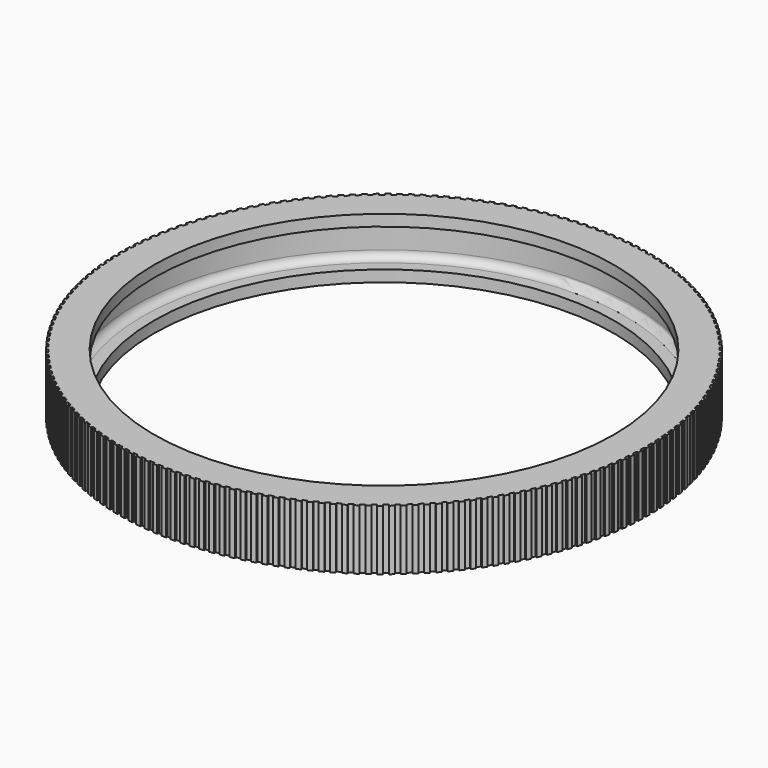
from build123d import *

# Parameters (mm, degrees)
F2_R     = 1
F4_DEPTH = 8


with BuildPart() as f1:
    # F0 (on Front) → F1 (revolve)
    with BuildSketch(Plane.XZ):
        Polygon((35, 8), (30.5, 8), (30.5, 6.5), (33, 6.5), (33, 1.5), (30.5, 1.5), (30.5, 0), (35, 0), align=None)
    revolve(axis=Axis((0, 0, 5), (0, 0, 1)))

    # F2
    f2_edges = [f1.edges().sort_by_distance(p)[0] for p in [
        (-33, 0, 6.5),
        (-33, 0, 1.5),
    ]]
    fillet(f2_edges, radius=F2_R)

    # F3 (on face) → F4 (cut, through all)
    with BuildSketch(Plane.XY.offset(8)):
        with BuildLine():
            Line((0.9096489537, 34.7380920429), (0.9161931908, 34.9880063741))
            ThreePointArc((0.9161931908, 34.9880063741), (0.6108342253, 34.9946693305), (0.3054287424, 34.9986673072))
            Line((0.3054287424, 34.9986673072), (0.3032471086, 34.7486768265))
            ThreePointArc((0.3032471086, 34.7486768265), (0.6064711237, 34.7447074067), (0.9096489537, 34.7380920429))
        make_face()
        with BuildLine():
            Line((2.1214367488, 34.6851842452), (2.1366988837, 34.9347179448))
            ThreePointArc((2.1366988837, 34.9347179448), (1.8317584685, 34.9520337164), (1.5266785578, 34.9666877554))
            Line((1.5266785578, 34.9666877554), (1.5157737109, 34.7169257))
            ThreePointArc((1.5157737109, 34.7169257), (1.8186744794, 34.7023763327), (2.1214367488, 34.6851842452))
        make_face()
        with BuildLine():
            Line((3.3306399001, 34.5900178933), (3.3546013382, 34.8388669429))
            ThreePointArc((3.3546013382, 34.8388669429), (3.0504509962, 34.8668144332), (2.7460683505, 34.8921066807))
            Line((2.7460683505, 34.8921066807), (2.7264535765, 34.6428773472))
            ThreePointArc((2.7264535765, 34.6428773472), (3.0286620605, 34.6177657587), (3.3306399001, 34.5900178933))
        make_face()
        with BuildLine():
            Line((4.5357851796, 34.4527089327), (4.5684167277, 34.7005701481))
            ThreePointArc((4.5684167277, 34.7005701481), (4.2654270192, 34.7391153074), (3.9621124819, 34.7750149487))
            Line((3.9621124819, 34.7750149487), (3.9338116784, 34.5266219848))
            ThreePointArc((3.9338116784, 34.5266219848), (4.2349596833, 34.4909787695), (4.5357851796, 34.4527089327))
        make_face()
        with BuildLine():
            Line((5.7354043037, 34.2734246534), (5.7766662051, 34.5199960538))
            ThreePointArc((5.7766662051, 34.5199960538), (5.4752062764, 34.5690919208), (5.1733293895, 34.6155552177))
            Line((5.1733293895, 34.6155552177), (5.1363770368, 34.3683012518))
            ThreePointArc((5.1363770368, 34.3683012518), (5.4360976601, 34.3221698357), (5.7354043037, 34.2734246534))
        make_face()
        with BuildLine():
            Line((6.928035721, 34.0523834856), (6.9778777046, 34.2973646617))
            ThreePointArc((6.9778777046, 34.2973646617), (6.6783148382, 34.3569514207), (6.3782433922, 34.4139217647))
            Line((6.3782433922, 34.4139217647), (6.3326845109, 34.1681080378))
            ThreePointArc((6.3326845109, 34.1681080378), (6.6306125893, 34.1115446248), (6.928035721, 34.0523834856))
        make_face()
        with BuildLine():
            Line((8.112226394, 33.7898547338), (8.170587735, 34.0329472139))
            ThreePointArc((8.170587735, 34.0329472139), (7.873286902, 34.1029522675), (7.5753864878, 34.1703602492))
            Line((7.5753864878, 34.1703602492), (7.5212765843, 33.9262862474))
            ThreePointArc((7.5212765843, 33.9262862474), (7.8170491384, 33.8593597513), (8.112226394, 33.7898547338))
        make_face()
        with BuildLine():
            Line((9.2865335687, 33.486158249), (9.3533431627, 33.7270658623))
            ThreePointArc((9.3533431627, 33.7270658623), (9.0586665786, 33.8074039201), (8.7633001419, 33.8851674132))
            Line((8.7633001419, 33.8851674132), (8.7007051409, 33.6431305031))
            ThreePointArc((8.7007051409, 33.6431305031), (8.9939618173, 33.5659224635), (9.2865335687, 33.486158249))
        make_face()
        with BuildLine():
            Line((10.4495265328, 33.1416640385), (10.5247029826, 33.3800932762))
            ThreePointArc((10.5247029826, 33.3800932762), (10.2330096653, 33.4706664587), (9.9405370646, 33.5586907204))
            Line((9.9405370646, 33.5586907204), (9.8695332285, 33.3189857867))
            ThreePointArc((9.8695332285, 33.3189857867), (10.1599167391, 33.2315902697), (10.4495265328, 33.1416640385))
        make_face()
        with BuildLine():
            Line((11.5997883584, 32.7567918155), (11.6832400732, 32.9924521882))
            ThreePointArc((11.6832400732, 32.9924521882), (11.394885406, 33.093150146), (11.1056629742, 33.1913279322))
            Line((11.1056629742, 33.1913279322), (11.0263368101, 32.9542470184))
            ThreePointArc((11.0263368101, 32.9542470184), (11.3134933674, 32.8567705021), (11.5997883584, 32.7567918155))
        make_face()
        with BuildLine():
            Line((12.7359176287, 32.3320104874), (12.8275429354, 32.5646148794))
            ThreePointArc((12.8275429354, 32.5646148794), (12.5428782341, 32.6753149274), (12.2572583441, 32.7835266237))
            Line((12.2572583441, 32.7835266237), (12.1697064988, 32.5493585764))
            ThreePointArc((12.1697064988, 32.5493585764), (12.4532862467, 32.4419198208), (12.7359176287, 32.3320104874))
        make_face()
        with BuildLine():
            Line((13.8565301452, 31.8678375849), (13.9562174124, 32.0971026035))
            ThreePointArc((13.9562174124, 32.0971026035), (13.6755894971, 32.2176698708), (13.3939201328, 32.3357836379))
            Line((13.3939201328, 32.3357836379), (13.2982492747, 32.1048137548))
            ThreePointArc((13.2982492747, 32.1048137548), (13.577906715, 31.9875436575), (13.8565301452, 31.8678375849))
        make_face()
        with BuildLine():
            Line((14.9602606141, 31.3648386312), (15.0678883883, 31.5904849522))
            ThreePointArc((15.0678883883, 31.5904849522), (14.7916391609, 31.7207725463), (14.514263493, 31.8486444807))
            Line((14.514263493, 31.8486444807), (14.4105901823, 31.621154163))
            ThreePointArc((14.4105901823, 31.621154163), (14.6859845955, 31.4941955995), (14.9602606141, 31.3648386312))
        make_face()
        with BuildLine():
            Line((16.0457643099, 30.8236264529), (16.1612014632, 31.0453791612))
            ThreePointArc((16.1612014632, 31.0453791612), (15.8896674909, 31.1852283466), (15.6169234588, 31.3227026561))
            Line((15.6169234588, 31.3227026561), (15.5053740056, 31.0989690657))
            ThreePointArc((15.5053740056, 31.0989690657), (15.7761698659, 30.9624767155), (16.0457643099, 30.8236264529))
        make_face()
        with BuildLine():
            Line((17.1117187136, 30.2448604339), (17.2348246036, 30.4624493579))
            ThreePointArc((17.2348246036, 30.4624493579), (16.9683367086, 30.6116897499), (16.7005566091, 30.7585989432))
            Line((16.7005566091, 30.7585989432), (16.581266919, 30.538894665))
            ThreePointArc((16.581266919, 30.538894665), (16.8471343036, 30.3930348231), (17.1117187136, 30.2448604339))
        make_face()
        with BuildLine():
            Line((18.1568251239, 29.6292457113), (18.2874497651, 29.8424057524))
            ThreePointArc((18.2874497651, 29.8424057524), (18.0263326219, 30.0008555246), (17.7638427036, 30.1570206155))
            Line((17.7638427036, 30.1570206155), (17.6369581129, 29.9416133253))
            ThreePointArc((17.6369581129, 29.9416133253), (17.8975731031, 29.7865636994), (18.1568251239, 29.6292457113))
        make_face()
        with BuildLine():
            Line((19.1798102396, 28.9775323168), (19.3177944859, 29.1860037723))
            ThreePointArc((19.3177944859, 29.1860037723), (19.0623662255, 29.3534698781), (18.8054862921, 29.5187006034))
            Line((18.8054862921, 29.5187006034), (18.6711613901, 29.307852742))
            ThreePointArc((18.6711613901, 29.307852742), (18.9262064668, 29.1438022361), (19.1798102396, 28.9775323168))
        make_face()
        with BuildLine():
            Line((20.179427711, 28.2905142629), (20.3246034499, 28.4940431425))
            ThreePointArc((20.3246034499, 28.4940431425), (20.0751752723, 28.6703215501), (19.8242182924, 28.8444166018))
            Line((19.8242182924, 28.8444166018), (19.6826167331, 28.6383850546))
            ThreePointArc((19.6826167331, 28.6383850546), (19.9317811632, 28.465533539), (20.179427711, 28.2905142629))
        make_face()
        with BuildLine():
            Line((21.1544596581, 27.5690285751), (21.3066500153, 27.7673669102))
            ThreePointArc((21.3066500153, 27.7673669102), (21.0635258103, 27.9522428517), (20.8187975363, 28.1349901216))
            Line((20.8187975363, 28.1349901216), (20.6700918396, 27.9340259064))
            ThreePointArc((20.6700918396, 27.9340259064), (20.9130720545, 27.7525839741), (21.1544596581, 27.5690285751))
        make_face()
        with BuildLine():
            Line((22.1037181547, 26.8139542727), (22.2627377097, 27.0068604186))
            ThreePointArc((22.2627377097, 27.0068604186), (22.0262136867, 27.200108651), (21.7880122823, 27.3912854898))
            Line((21.7880122823, 27.3912854898), (21.6323836232, 27.1956334506))
            ThreePointArc((21.6323836232, 27.1956334506), (21.868883589, 27.0058221606), (22.1037181547, 26.8139542727))
        make_face()
        with BuildLine():
            Line((23.0260466755, 26.0262112974), (23.1917016875, 26.2134502276))
            ThreePointArc((23.1917016875, 26.2134502276), (22.9620660147, 26.4148353078), (22.7306816916, 26.614208796))
            Line((22.7306816916, 26.614208796), (22.5683196795, 26.4241073046))
            ThreePointArc((22.5683196795, 26.4241073046), (22.7980512574, 26.2261579127), (23.0260466755, 26.0262112974))
        make_face()
        with BuildLine():
            Line((23.9203215054, 25.2067593927), (24.0924101493, 25.3881029854))
            ThreePointArc((24.0924101493, 25.3881029854), (23.8699426022, 25.5973795567), (23.6456572665, 25.8047067884))
            Line((23.6456572665, 25.8047067884), (23.4767597146, 25.6203874541))
            ThreePointArc((23.4767597146, 25.6203874541), (23.6994430122, 25.4145411313), (23.9203215054, 25.2067593927))
        make_face()
        with BuildLine():
            Line((24.7854531081, 24.3565969344), (24.9637657204, 24.5318242505))
            ThreePointArc((24.9637657204, 24.5318242505), (24.7487373415, 24.7487373415), (24.5318242505, 24.9637657204))
            Line((24.5318242505, 24.9637657204), (24.3565969344, 24.7854531081))
            ThreePointArc((24.3565969344, 24.7854531081), (24.5719606462, 24.5719606462), (24.7854531081, 24.3565969344))
        make_face()
        with BuildLine():
            Line((25.6203874542, 23.4767597146), (25.8047067884, 23.6456572665))
            ThreePointArc((25.8047067884, 23.6456572665), (25.5973795567, 23.8699426022), (25.3881029854, 24.0924101493))
            Line((25.3881029854, 24.0924101493), (25.2067593927, 23.9203215054))
            ThreePointArc((25.2067593927, 23.9203215054), (25.4145411313, 23.6994430122), (25.6203874542, 23.4767597146))
        make_face()
        with BuildLine():
            Line((26.4241073046, 22.5683196795), (26.614208796, 22.7306816916))
            ThreePointArc((26.614208796, 22.7306816916), (26.4148353078, 22.9620660147), (26.2134502276, 23.1917016875))
            Line((26.2134502276, 23.1917016875), (26.0262112974, 23.0260466755))
            ThreePointArc((26.0262112974, 23.0260466755), (26.2261579127, 22.7980512574), (26.4241073046, 22.5683196795))
        make_face()
        with BuildLine():
            Line((27.1956334506, 21.6323836232), (27.3912854898, 21.7880122823))
            ThreePointArc((27.3912854898, 21.7880122823), (27.200108651, 22.0262136867), (27.0068604186, 22.2627377097))
            Line((27.0068604186, 22.2627377097), (26.8139542727, 22.1037181546))
            ThreePointArc((26.8139542727, 22.1037181546), (27.0058221606, 21.868883589), (27.1956334506, 21.6323836232))
        make_face()
        with BuildLine():
            Line((27.9340259064, 20.6700918396), (28.1349901216, 20.8187975363))
            ThreePointArc((28.1349901216, 20.8187975363), (27.9522428517, 21.0635258103), (27.7673669102, 21.3066500153))
            Line((27.7673669102, 21.3066500153), (27.5690285751, 21.154459658))
            ThreePointArc((27.5690285751, 21.154459658), (27.7525839741, 20.9130720545), (27.9340259064, 20.6700918396))
        make_face()
        with BuildLine():
            Line((28.6383850546, 19.6826167331), (28.8444166018, 19.8242182924))
            ThreePointArc((28.8444166018, 19.8242182924), (28.6703215501, 20.0751752723), (28.4940431425, 20.3246034499))
            Line((28.4940431425, 20.3246034499), (28.2905142629, 20.179427711))
            ThreePointArc((28.2905142629, 20.179427711), (28.465533539, 19.9317811632), (28.6383850546, 19.6826167331))
        make_face()
        with BuildLine():
            Line((29.307852742, 18.67116139), (29.5187006034, 18.8054862921))
            ThreePointArc((29.5187006034, 18.8054862921), (29.3534698781, 19.0623662255), (29.1860037723, 19.3177944859))
            Line((29.1860037723, 19.3177944859), (28.9775323168, 19.1798102396))
            ThreePointArc((28.9775323168, 19.1798102396), (29.1438022361, 18.9262064668), (29.307852742, 18.67116139))
        make_face()
        with BuildLine():
            Line((29.9416133253, 17.6369581129), (30.1570206155, 17.7638427036))
            ThreePointArc((30.1570206155, 17.7638427036), (30.0008555246, 18.0263326218), (29.8424057524, 18.2874497651))
            Line((29.8424057524, 18.2874497651), (29.6292457113, 18.1568251239))
            ThreePointArc((29.6292457113, 18.1568251239), (29.7865636994, 17.8975731031), (29.9416133253, 17.6369581129))
        make_face()
        with BuildLine():
            Line((30.538894665, 16.581266919), (30.7585989432, 16.7005566091))
            ThreePointArc((30.7585989432, 16.7005566091), (30.6116897499, 16.9683367086), (30.4624493579, 17.2348246036))
            Line((30.4624493579, 17.2348246036), (30.2448604339, 17.1117187136))
            ThreePointArc((30.2448604339, 17.1117187136), (30.3930348231, 16.8471343036), (30.538894665, 16.581266919))
        make_face()
        with BuildLine():
            Line((31.0989690657, 15.5053740056), (31.3227026561, 15.6169234588))
            ThreePointArc((31.3227026561, 15.6169234588), (31.1852283466, 15.8896674909), (31.0453791612, 16.1612014632))
            Line((31.0453791612, 16.1612014632), (30.8236264529, 16.0457643099))
            ThreePointArc((30.8236264529, 16.0457643099), (30.9624767155, 15.7761698659), (31.0989690657, 15.5053740056))
        make_face()
        with BuildLine():
            Line((31.621154163, 14.4105901823), (31.8486444807, 14.514263493))
            ThreePointArc((31.8486444807, 14.514263493), (31.7207725463, 14.7916391609), (31.5904849522, 15.0678883883))
            Line((31.5904849522, 15.0678883883), (31.3648386312, 14.9602606141))
            ThreePointArc((31.3648386312, 14.9602606141), (31.4941955995, 14.6859845955), (31.621154163, 14.4105901823))
        make_face()
        with BuildLine():
            Line((32.1048137548, 13.2982492747), (32.3357836379, 13.3939201328))
            ThreePointArc((32.3357836379, 13.3939201328), (32.2176698708, 13.6755894971), (32.0971026035, 13.9562174124))
            Line((32.0971026035, 13.9562174124), (31.8678375849, 13.8565301451))
            ThreePointArc((31.8678375849, 13.8565301451), (31.9875436575, 13.577906715), (32.1048137548, 13.2982492747))
        make_face()
        with BuildLine():
            Line((32.5493585764, 12.1697064988), (32.7835266237, 12.2572583441))
            ThreePointArc((32.7835266237, 12.2572583441), (32.6753149274, 12.5428782341), (32.5646148794, 12.8275429353))
            Line((32.5646148794, 12.8275429353), (32.3320104874, 12.7359176287))
            ThreePointArc((32.3320104874, 12.7359176287), (32.4419198208, 12.4532862467), (32.5493585764, 12.1697064988))
        make_face()
        with BuildLine():
            Line((32.9542470184, 11.0263368101), (33.1913279322, 11.1056629742))
            ThreePointArc((33.1913279322, 11.1056629742), (33.093150146, 11.394885406), (32.9924521882, 11.6832400732))
            Line((32.9924521882, 11.6832400732), (32.7567918155, 11.5997883584))
            ThreePointArc((32.7567918155, 11.5997883584), (32.8567705021, 11.3134933674), (32.9542470184, 11.0263368101))
        make_face()
        with BuildLine():
            Line((33.3189857867, 9.8695332285), (33.5586907204, 9.9405370646))
            ThreePointArc((33.5586907204, 9.9405370646), (33.4706664587, 10.2330096653), (33.3800932762, 10.5247029826))
            Line((33.3800932762, 10.5247029826), (33.1416640385, 10.4495265328))
            ThreePointArc((33.1416640385, 10.4495265328), (33.2315902697, 10.1599167391), (33.3189857867, 9.8695332285))
        make_face()
        with BuildLine():
            Line((33.6431305031, 8.7007051409), (33.8851674132, 8.7633001419))
            ThreePointArc((33.8851674132, 8.7633001419), (33.8074039201, 9.0586665786), (33.7270658623, 9.3533431627))
            Line((33.7270658623, 9.3533431627), (33.486158249, 9.2865335687))
            ThreePointArc((33.486158249, 9.2865335687), (33.5659224635, 8.9939618173), (33.6431305031, 8.7007051409))
        make_face()
        with BuildLine():
            Line((33.9262862474, 7.5212765843), (34.1703602492, 7.5753864878))
            ThreePointArc((34.1703602492, 7.5753864878), (34.1029522675, 7.873286902), (34.0329472139, 8.170587735))
            Line((34.0329472139, 8.170587735), (33.7898547338, 8.112226394))
            ThreePointArc((33.7898547338, 8.112226394), (33.8593597513, 7.8170491384), (33.9262862474, 7.5212765843))
        make_face()
        with BuildLine():
            Line((34.1681080378, 6.3326845108), (34.4139217647, 6.3782433922))
            ThreePointArc((34.4139217647, 6.3782433922), (34.3569514207, 6.6783148382), (34.2973646617, 6.9778777046))
            Line((34.2973646617, 6.9778777046), (34.0523834856, 6.928035721))
            ThreePointArc((34.0523834856, 6.928035721), (34.1115446248, 6.6306125893), (34.1681080378, 6.3326845108))
        make_face()
        with BuildLine():
            Line((34.3683012518, 5.1363770367), (34.6155552177, 5.1733293895))
            ThreePointArc((34.6155552177, 5.1733293895), (34.5690919208, 5.4752062764), (34.5199960538, 5.7766662051))
            Line((34.5199960538, 5.7766662051), (34.2734246534, 5.7354043037))
            ThreePointArc((34.2734246534, 5.7354043037), (34.3221698357, 5.4360976601), (34.3683012518, 5.1363770367))
        make_face()
        with BuildLine():
            Line((34.5266219848, 3.9338116784), (34.7750149487, 3.9621124819))
            ThreePointArc((34.7750149487, 3.9621124819), (34.7391153074, 4.2654270192), (34.7005701481, 4.5684167277))
            Line((34.7005701481, 4.5684167277), (34.4527089327, 4.5357851796))
            ThreePointArc((34.4527089327, 4.5357851796), (34.4909787695, 4.2349596833), (34.5266219848, 3.9338116784))
        make_face()
        with BuildLine():
            Line((34.6428773472, 2.7264535765), (34.8921066807, 2.7460683505))
            ThreePointArc((34.8921066807, 2.7460683505), (34.8668144332, 3.0504509962), (34.8388669428, 3.3546013382))
            Line((34.8388669428, 3.3546013382), (34.5900178933, 3.3306399001))
            ThreePointArc((34.5900178933, 3.3306399001), (34.6177657587, 3.0286620605), (34.6428773472, 2.7264535765))
        make_face()
        with BuildLine():
            Line((34.7169257, 1.5157737109), (34.9666877554, 1.5266785578))
            ThreePointArc((34.9666877554, 1.5266785578), (34.9520337164, 1.8317584685), (34.9347179448, 2.1366988837))
            Line((34.9347179448, 2.1366988837), (34.6851842452, 2.1214367488))
            ThreePointArc((34.6851842452, 2.1214367488), (34.7023763327, 1.8186744794), (34.7169257, 1.5157737109))
        make_face()
        with BuildLine():
            Line((34.7486768265, 0.3032471086), (34.9986673072, 0.3054287424))
            ThreePointArc((34.9986673072, 0.3054287424), (34.9946693305, 0.6108342253), (34.9880063741, 0.9161931908))
            Line((34.9880063741, 0.9161931908), (34.7380920429, 0.9096489537))
            ThreePointArc((34.7380920429, 0.9096489537), (34.7447074067, 0.6064711237), (34.7486768265, 0.3032471086))
        make_face()
        with BuildLine():
            Line((34.7380920429, -0.9096489537), (34.9880063741, -0.9161931908))
            ThreePointArc((34.9880063741, -0.9161931908), (34.9946693305, -0.6108342253), (34.9986673072, -0.3054287424))
            Line((34.9986673072, -0.3054287424), (34.7486768265, -0.3032471086))
            ThreePointArc((34.7486768265, -0.3032471086), (34.7447074067, -0.6064711237), (34.7380920429, -0.9096489537))
        make_face()
        with BuildLine():
            Line((34.6851842452, -2.1214367488), (34.9347179448, -2.1366988837))
            ThreePointArc((34.9347179448, -2.1366988837), (34.9520337164, -1.8317584685), (34.9666877554, -1.5266785578))
            Line((34.9666877554, -1.5266785578), (34.7169257, -1.515773711))
            ThreePointArc((34.7169257, -1.5157737109), (34.7023763327, -1.8186744794), (34.6851842452, -2.1214367488))
        make_face()
        with BuildLine():
            Line((34.5900178933, -3.3306399001), (34.8388669428, -3.3546013382))
            ThreePointArc((34.8388669428, -3.3546013382), (34.8668144332, -3.0504509962), (34.8921066807, -2.7460683505))
            Line((34.8921066807, -2.7460683505), (34.6428773472, -2.7264535765))
            ThreePointArc((34.6428773472, -2.7264535765), (34.6177657587, -3.0286620605), (34.5900178933, -3.3306399001))
        make_face()
        with BuildLine():
            Line((34.4527089327, -4.5357851797), (34.7005701481, -4.5684167277))
            ThreePointArc((34.7005701481, -4.5684167277), (34.7391153074, -4.2654270192), (34.7750149487, -3.9621124819))
            Line((34.7750149487, -3.9621124819), (34.5266219848, -3.9338116784))
            ThreePointArc((34.5266219848, -3.9338116784), (34.4909787695, -4.2349596833), (34.4527089327, -4.5357851797))
        make_face()
        with BuildLine():
            Line((34.2734246534, -5.7354043037), (34.5199960538, -5.7766662051))
            ThreePointArc((34.5199960538, -5.7766662051), (34.5690919208, -5.4752062764), (34.6155552177, -5.1733293895))
            Line((34.6155552177, -5.1733293895), (34.3683012518, -5.1363770368))
            ThreePointArc((34.3683012518, -5.1363770368), (34.3221698357, -5.4360976602), (34.2734246534, -5.7354043037))
        make_face()
        with BuildLine():
            Line((34.0523834856, -6.928035721), (34.2973646617, -6.9778777046))
            ThreePointArc((34.2973646617, -6.9778777046), (34.3569514207, -6.6783148382), (34.4139217647, -6.3782433922))
            Line((34.4139217647, -6.3782433922), (34.1681080378, -6.3326845109))
            ThreePointArc((34.1681080378, -6.3326845109), (34.1115446248, -6.6306125893), (34.0523834856, -6.928035721))
        make_face()
        with BuildLine():
            Line((33.7898547338, -8.112226394), (34.0329472139, -8.170587735))
            ThreePointArc((34.0329472139, -8.170587735), (34.1029522675, -7.873286902), (34.1703602492, -7.5753864878))
            Line((34.1703602492, -7.5753864878), (33.9262862474, -7.5212765844))
            ThreePointArc((33.9262862474, -7.5212765844), (33.8593597513, -7.8170491385), (33.7898547338, -8.112226394))
        make_face()
        with BuildLine():
            Line((33.486158249, -9.2865335687), (33.7270658623, -9.3533431627))
            ThreePointArc((33.7270658623, -9.3533431627), (33.8074039201, -9.0586665786), (33.8851674132, -8.7633001419))
            Line((33.8851674132, -8.7633001419), (33.6431305031, -8.7007051409))
            ThreePointArc((33.6431305031, -8.7007051409), (33.5659224635, -8.9939618173), (33.486158249, -9.2865335687))
        make_face()
        with BuildLine():
            Line((33.1416640385, -10.4495265328), (33.3800932762, -10.5247029827))
            ThreePointArc((33.3800932762, -10.5247029827), (33.4706664587, -10.2330096653), (33.5586907204, -9.9405370646))
            Line((33.5586907204, -9.9405370646), (33.3189857867, -9.8695332285))
            ThreePointArc((33.3189857867, -9.8695332285), (33.2315902697, -10.1599167391), (33.1416640385, -10.4495265328))
        make_face()
        with BuildLine():
            Line((32.7567918154, -11.5997883584), (32.9924521882, -11.6832400732))
            ThreePointArc((32.9924521882, -11.6832400732), (33.093150146, -11.394885406), (33.1913279322, -11.1056629742))
            Line((33.1913279322, -11.1056629742), (32.9542470184, -11.0263368101))
            ThreePointArc((32.9542470184, -11.0263368101), (32.8567705021, -11.3134933674), (32.7567918154, -11.5997883584))
        make_face()
        with BuildLine():
            Line((32.3320104874, -12.7359176287), (32.5646148794, -12.8275429354))
            ThreePointArc((32.5646148794, -12.8275429354), (32.6753149274, -12.5428782341), (32.7835266237, -12.2572583441))
            Line((32.7835266237, -12.2572583441), (32.5493585764, -12.1697064988))
            ThreePointArc((32.5493585764, -12.1697064988), (32.4419198208, -12.4532862467), (32.3320104874, -12.7359176287))
        make_face()
        with BuildLine():
            Line((31.8678375849, -13.8565301452), (32.0971026035, -13.9562174124))
            ThreePointArc((32.0971026035, -13.9562174124), (32.2176698708, -13.6755894971), (32.3357836379, -13.3939201328))
            Line((32.3357836379, -13.3939201328), (32.1048137548, -13.2982492747))
            ThreePointArc((32.1048137548, -13.2982492747), (31.9875436575, -13.577906715), (31.8678375849, -13.8565301452))
        make_face()
        with BuildLine():
            Line((31.3648386312, -14.9602606141), (31.5904849522, -15.0678883883))
            ThreePointArc((31.5904849522, -15.0678883883), (31.7207725463, -14.7916391609), (31.8486444807, -14.514263493))
            Line((31.8486444807, -14.514263493), (31.621154163, -14.4105901823))
            ThreePointArc((31.621154163, -14.4105901823), (31.4941955995, -14.6859845955), (31.3648386312, -14.9602606141))
        make_face()
        with BuildLine():
            Line((30.8236264529, -16.0457643099), (31.0453791612, -16.1612014632))
            ThreePointArc((31.0453791612, -16.1612014632), (31.1852283466, -15.8896674909), (31.3227026561, -15.6169234588))
            Line((31.3227026561, -15.6169234588), (31.0989690657, -15.5053740056))
            ThreePointArc((31.0989690657, -15.5053740056), (30.9624767155, -15.776169866), (30.8236264529, -16.0457643099))
        make_face()
        with BuildLine():
            Line((30.2448604339, -17.1117187136), (30.4624493579, -17.2348246036))
            ThreePointArc((30.4624493579, -17.2348246036), (30.6116897499, -16.9683367086), (30.7585989432, -16.7005566091))
            Line((30.7585989432, -16.7005566091), (30.538894665, -16.581266919))
            ThreePointArc((30.538894665, -16.581266919), (30.3930348231, -16.8471343036), (30.2448604339, -17.1117187136))
        make_face()
        with BuildLine():
            Line((29.6292457113, -18.1568251239), (29.8424057524, -18.2874497651))
            ThreePointArc((29.8424057524, -18.2874497651), (30.0008555246, -18.0263326219), (30.1570206154, -17.7638427036))
            Line((30.1570206154, -17.7638427036), (29.9416133253, -17.6369581129))
            ThreePointArc((29.9416133253, -17.6369581129), (29.7865636994, -17.8975731031), (29.6292457113, -18.1568251239))
        make_face()
        with BuildLine():
            Line((28.9775323168, -19.1798102396), (29.1860037723, -19.3177944859))
            ThreePointArc((29.1860037723, -19.3177944859), (29.3534698781, -19.0623662255), (29.5187006034, -18.8054862921))
            Line((29.5187006034, -18.8054862921), (29.307852742, -18.6711613901))
            ThreePointArc((29.307852742, -18.6711613901), (29.1438022361, -18.9262064668), (28.9775323168, -19.1798102396))
        make_face()
        with BuildLine():
            Line((28.2905142629, -20.179427711), (28.4940431425, -20.3246034499))
            ThreePointArc((28.4940431425, -20.3246034499), (28.6703215501, -20.0751752723), (28.8444166018, -19.8242182924))
            Line((28.8444166018, -19.8242182924), (28.6383850546, -19.6826167331))
            ThreePointArc((28.6383850546, -19.6826167331), (28.465533539, -19.9317811632), (28.2905142629, -20.179427711))
        make_face()
        with BuildLine():
            Line((27.5690285751, -21.1544596581), (27.7673669102, -21.3066500153))
            ThreePointArc((27.7673669102, -21.3066500153), (27.9522428516, -21.0635258103), (28.1349901216, -20.8187975363))
            Line((28.1349901216, -20.8187975363), (27.9340259064, -20.6700918396))
            ThreePointArc((27.9340259064, -20.6700918396), (27.7525839741, -20.9130720545), (27.5690285751, -21.1544596581))
        make_face()
        with BuildLine():
            Line((26.8139542727, -22.1037181547), (27.0068604186, -22.2627377097))
            ThreePointArc((27.0068604186, -22.2627377097), (27.200108651, -22.0262136867), (27.3912854898, -21.7880122823))
            Line((27.3912854898, -21.7880122823), (27.1956334506, -21.6323836232))
            ThreePointArc((27.1956334506, -21.6323836232), (27.0058221606, -21.868883589), (26.8139542727, -22.1037181547))
        make_face()
        with BuildLine():
            Line((26.0262112974, -23.0260466755), (26.2134502276, -23.1917016876))
            ThreePointArc((26.2134502276, -23.1917016876), (26.4148353078, -22.9620660147), (26.614208796, -22.7306816916))
            Line((26.614208796, -22.7306816916), (26.4241073046, -22.5683196795))
            ThreePointArc((26.4241073046, -22.5683196795), (26.2261579127, -22.7980512574), (26.0262112974, -23.0260466755))
        make_face()
        with BuildLine():
            Line((25.2067593927, -23.9203215054), (25.3881029854, -24.0924101493))
            ThreePointArc((25.3881029854, -24.0924101493), (25.5973795567, -23.8699426022), (25.8047067883, -23.6456572666))
            Line((25.8047067883, -23.6456572666), (25.6203874541, -23.4767597146))
            ThreePointArc((25.6203874541, -23.4767597146), (25.4145411313, -23.6994430122), (25.2067593927, -23.9203215054))
        make_face()
        with BuildLine():
            Line((24.3565969344, -24.7854531081), (24.5318242505, -24.9637657204))
            ThreePointArc((24.5318242505, -24.9637657204), (24.7487373415, -24.7487373415), (24.9637657204, -24.5318242505))
            Line((24.9637657204, -24.5318242505), (24.7854531081, -24.3565969344))
            ThreePointArc((24.7854531081, -24.3565969344), (24.5719606462, -24.5719606462), (24.3565969344, -24.7854531081))
        make_face()
        with BuildLine():
            Line((23.4767597146, -25.6203874542), (23.6456572665, -25.8047067884))
            ThreePointArc((23.6456572665, -25.8047067884), (23.8699426022, -25.5973795567), (24.0924101493, -25.3881029854))
            Line((24.0924101493, -25.3881029854), (23.9203215053, -25.2067593927))
            ThreePointArc((23.9203215054, -25.2067593927), (23.6994430122, -25.4145411313), (23.4767597146, -25.6203874542))
        make_face()
        with BuildLine():
            Line((22.5683196795, -26.4241073046), (22.7306816915, -26.614208796))
            ThreePointArc((22.7306816915, -26.614208796), (22.9620660147, -26.4148353078), (23.1917016875, -26.2134502276))
            Line((23.1917016875, -26.2134502276), (23.0260466755, -26.0262112974))
            ThreePointArc((23.0260466755, -26.0262112974), (22.7980512574, -26.2261579127), (22.5683196795, -26.4241073046))
        make_face()
        with BuildLine():
            Line((21.6323836231, -27.1956334506), (21.7880122823, -27.3912854898))
            ThreePointArc((21.7880122823, -27.3912854898), (22.0262136867, -27.200108651), (22.2627377097, -27.0068604186))
            Line((22.2627377097, -27.0068604186), (22.1037181546, -26.8139542727))
            ThreePointArc((22.1037181546, -26.8139542727), (21.868883589, -27.0058221606), (21.6323836231, -27.1956334506))
        make_face()
        with BuildLine():
            Line((20.6700918396, -27.9340259065), (20.8187975363, -28.1349901216))
            ThreePointArc((20.8187975363, -28.1349901216), (21.0635258103, -27.9522428517), (21.3066500153, -27.7673669102))
            Line((21.3066500153, -27.7673669102), (21.154459658, -27.5690285751))
            ThreePointArc((21.154459658, -27.5690285751), (20.9130720545, -27.7525839741), (20.6700918396, -27.9340259065))
        make_face()
        with BuildLine():
            Line((19.6826167331, -28.6383850546), (19.8242182924, -28.8444166018))
            ThreePointArc((19.8242182924, -28.8444166018), (20.0751752723, -28.6703215501), (20.3246034499, -28.4940431425))
            Line((20.3246034499, -28.4940431425), (20.1794277109, -28.2905142629))
            ThreePointArc((20.1794277109, -28.2905142629), (19.9317811632, -28.465533539), (19.6826167331, -28.6383850546))
        make_face()
        with BuildLine():
            Line((18.67116139, -29.307852742), (18.8054862921, -29.5187006035))
            ThreePointArc((18.8054862921, -29.5187006035), (19.0623662255, -29.3534698781), (19.3177944859, -29.1860037724))
            Line((19.3177944859, -29.1860037724), (19.1798102396, -28.9775323168))
            ThreePointArc((19.1798102396, -28.9775323168), (18.9262064668, -29.1438022361), (18.67116139, -29.307852742))
        make_face()
        with BuildLine():
            Line((17.6369581129, -29.9416133253), (17.7638427036, -30.1570206155))
            ThreePointArc((17.7638427036, -30.1570206155), (18.0263326218, -30.0008555246), (18.2874497651, -29.8424057524))
            Line((18.287449765, -29.8424057524), (18.1568251239, -29.6292457113))
            ThreePointArc((18.1568251239, -29.6292457113), (17.8975731031, -29.7865636994), (17.6369581129, -29.9416133253))
        make_face()
        with BuildLine():
            Line((16.581266919, -30.538894665), (16.7005566091, -30.7585989432))
            ThreePointArc((16.7005566091, -30.7585989432), (16.9683367086, -30.6116897499), (17.2348246036, -30.4624493579))
            Line((17.2348246036, -30.4624493579), (17.1117187136, -30.2448604339))
            ThreePointArc((17.1117187136, -30.2448604339), (16.8471343036, -30.3930348231), (16.581266919, -30.538894665))
        make_face()
        with BuildLine():
            Line((15.5053740056, -31.0989690657), (15.6169234588, -31.3227026561))
            ThreePointArc((15.6169234588, -31.3227026561), (15.8896674909, -31.1852283466), (16.1612014632, -31.0453791612))
            Line((16.1612014632, -31.0453791612), (16.0457643099, -30.8236264529))
            ThreePointArc((16.0457643099, -30.8236264529), (15.7761698659, -30.9624767155), (15.5053740056, -31.0989690657))
        make_face()
        with BuildLine():
            Line((14.4105901823, -31.621154163), (14.514263493, -31.8486444807))
            ThreePointArc((14.514263493, -31.8486444807), (14.7916391609, -31.7207725463), (15.0678883883, -31.5904849522))
            Line((15.0678883883, -31.5904849522), (14.9602606141, -31.3648386312))
            ThreePointArc((14.9602606141, -31.3648386312), (14.6859845955, -31.4941955995), (14.4105901823, -31.621154163))
        make_face()
        with BuildLine():
            Line((13.2982492747, -32.1048137548), (13.3939201328, -32.3357836379))
            ThreePointArc((13.3939201328, -32.3357836379), (13.6755894971, -32.2176698708), (13.9562174124, -32.0971026035))
            Line((13.9562174124, -32.0971026035), (13.8565301451, -31.8678375849))
            ThreePointArc((13.8565301451, -31.8678375849), (13.577906715, -31.9875436575), (13.2982492747, -32.1048137548))
        make_face()
        with BuildLine():
            Line((12.1697064988, -32.5493585764), (12.2572583441, -32.7835266237))
            ThreePointArc((12.2572583441, -32.7835266237), (12.5428782341, -32.6753149274), (12.8275429353, -32.5646148794))
            Line((12.8275429353, -32.5646148794), (12.7359176287, -32.3320104874))
            ThreePointArc((12.7359176287, -32.3320104874), (12.4532862467, -32.4419198208), (12.1697064988, -32.5493585764))
        make_face()
        with BuildLine():
            Line((11.0263368101, -32.9542470184), (11.1056629742, -33.1913279322))
            ThreePointArc((11.1056629742, -33.1913279322), (11.394885406, -33.093150146), (11.6832400732, -32.9924521882))
            Line((11.6832400732, -32.9924521882), (11.5997883584, -32.7567918155))
            ThreePointArc((11.5997883584, -32.7567918155), (11.3134933674, -32.8567705021), (11.0263368101, -32.9542470184))
        make_face()
        with BuildLine():
            Line((9.8695332285, -33.3189857867), (9.9405370646, -33.5586907204))
            ThreePointArc((9.9405370646, -33.5586907204), (10.2330096653, -33.4706664587), (10.5247029826, -33.3800932762))
            Line((10.5247029826, -33.3800932762), (10.4495265328, -33.1416640385))
            ThreePointArc((10.4495265328, -33.1416640385), (10.1599167391, -33.2315902697), (9.8695332285, -33.3189857867))
        make_face()
        with BuildLine():
            Line((8.7007051409, -33.6431305031), (8.7633001419, -33.8851674132))
            ThreePointArc((8.7633001419, -33.8851674132), (9.0586665786, -33.8074039201), (9.3533431627, -33.7270658623))
            Line((9.3533431627, -33.7270658623), (9.2865335687, -33.486158249))
            ThreePointArc((9.2865335687, -33.486158249), (8.9939618173, -33.5659224635), (8.7007051409, -33.6431305031))
        make_face()
        with BuildLine():
            Line((7.5212765843, -33.9262862474), (7.5753864878, -34.1703602492))
            ThreePointArc((7.5753864878, -34.1703602492), (7.873286902, -34.1029522675), (8.1705877349, -34.0329472139))
            Line((8.1705877349, -34.0329472139), (8.112226394, -33.7898547338))
            ThreePointArc((8.112226394, -33.7898547338), (7.8170491384, -33.8593597513), (7.5212765843, -33.9262862474))
        make_face()
        with BuildLine():
            Line((6.3326845108, -34.1681080378), (6.3782433922, -34.4139217647))
            ThreePointArc((6.3782433922, -34.4139217647), (6.6783148382, -34.3569514207), (6.9778777046, -34.2973646617))
            Line((6.9778777046, -34.2973646617), (6.928035721, -34.0523834856))
            ThreePointArc((6.928035721, -34.0523834856), (6.6306125893, -34.1115446248), (6.3326845108, -34.1681080378))
        make_face()
        with BuildLine():
            Line((5.1363770367, -34.3683012518), (5.1733293895, -34.6155552177))
            ThreePointArc((5.1733293895, -34.6155552177), (5.4752062764, -34.5690919208), (5.7766662051, -34.5199960538))
            Line((5.7766662051, -34.5199960538), (5.7354043036, -34.2734246534))
            ThreePointArc((5.7354043036, -34.2734246534), (5.4360976601, -34.3221698357), (5.1363770367, -34.3683012518))
        make_face()
        with BuildLine():
            Line((3.9338116784, -34.5266219848), (3.9621124819, -34.7750149487))
            ThreePointArc((3.9621124819, -34.7750149487), (4.2654270192, -34.7391153074), (4.5684167277, -34.7005701481))
            Line((4.5684167277, -34.7005701481), (4.5357851796, -34.4527089327))
            ThreePointArc((4.5357851796, -34.4527089327), (4.2349596833, -34.4909787695), (3.9338116784, -34.5266219848))
        make_face()
        with BuildLine():
            Line((2.7264535765, -34.6428773472), (2.7460683505, -34.8921066807))
            ThreePointArc((2.7460683505, -34.8921066807), (3.0504509962, -34.8668144332), (3.3546013382, -34.8388669429))
            Line((3.3546013382, -34.8388669429), (3.3306399001, -34.5900178933))
            ThreePointArc((3.3306399001, -34.5900178933), (3.0286620605, -34.6177657587), (2.7264535765, -34.6428773472))
        make_face()
        with BuildLine():
            Line((1.5157737109, -34.7169257), (1.5266785578, -34.9666877554))
            ThreePointArc((1.5266785578, -34.9666877554), (1.8317584685, -34.9520337164), (2.1366988837, -34.9347179448))
            Line((2.1366988837, -34.9347179448), (2.1214367488, -34.6851842452))
            ThreePointArc((2.1214367488, -34.6851842452), (1.8186744794, -34.7023763327), (1.5157737109, -34.7169257))
        make_face()
        with BuildLine():
            Line((0.3032471086, -34.7486768265), (0.3054287424, -34.9986673072))
            ThreePointArc((0.3054287424, -34.9986673072), (0.6108342253, -34.9946693305), (0.9161931908, -34.9880063741))
            Line((0.9161931908, -34.9880063741), (0.9096489537, -34.7380920429))
            ThreePointArc((0.9096489537, -34.7380920429), (0.6064711237, -34.7447074067), (0.3032471086, -34.7486768265))
        make_face()
        with BuildLine():
            ThreePointArc((-34.9880063741, 0.9161931908), (-34.9946693305, 0.6108342253), (-34.9986673072, 0.3054287424))
            Line((-34.9986673072, 0.3054287424), (-34.7486768265, 0.3032471086))
            ThreePointArc((-34.7486768265, 0.3032471086), (-34.7447074067, 0.6064711237), (-34.7380920429, 0.9096489537))
            Line((-34.7380920429, 0.9096489537), (-34.9880063741, 0.9161931908))
        make_face()
        with BuildLine():
            ThreePointArc((-34.9347179448, 2.1366988837), (-34.9520337164, 1.8317584685), (-34.9666877554, 1.5266785578))
            Line((-34.9666877554, 1.5266785578), (-34.7169257, 1.5157737109))
            ThreePointArc((-34.7169257, 1.5157737109), (-34.7023763327, 1.8186744794), (-34.6851842452, 2.1214367488))
            Line((-34.6851842452, 2.1214367488), (-34.9347179448, 2.1366988837))
        make_face()
        with BuildLine():
            ThreePointArc((-34.8388669428, 3.3546013382), (-34.8668144332, 3.0504509962), (-34.8921066807, 2.7460683505))
            Line((-34.8921066807, 2.7460683505), (-34.6428773472, 2.7264535765))
            ThreePointArc((-34.6428773472, 2.7264535765), (-34.6177657587, 3.0286620605), (-34.5900178933, 3.3306399001))
            Line((-34.5900178933, 3.3306399001), (-34.8388669428, 3.3546013382))
        make_face()
        with BuildLine():
            ThreePointArc((-34.9986673072, -0.3054287424), (-34.9946693305, -0.6108342253), (-34.9880063741, -0.9161931908))
            Line((-34.9880063741, -0.9161931908), (-34.7380920429, -0.9096489537))
            ThreePointArc((-34.7380920429, -0.9096489537), (-34.7447074067, -0.6064711237), (-34.7486768265, -0.3032471086))
            Line((-34.7486768265, -0.3032471086), (-34.9986673072, -0.3054287424))
        make_face()
        with BuildLine():
            Line((-34.7169257, -1.515773711), (-34.9666877554, -1.5266785578))
            ThreePointArc((-34.9666877554, -1.5266785578), (-34.9520337164, -1.8317584685), (-34.9347179448, -2.1366988837))
            Line((-34.9347179448, -2.1366988837), (-34.6851842452, -2.1214367488))
            ThreePointArc((-34.6851842452, -2.1214367488), (-34.7023763327, -1.8186744794), (-34.7169257, -1.5157737109))
        make_face()
        with BuildLine():
            ThreePointArc((-6.3782433922, 34.4139217647), (-6.6783148382, 34.3569514207), (-6.9778777046, 34.2973646617))
            Line((-6.9778777046, 34.2973646617), (-6.928035721, 34.0523834856))
            ThreePointArc((-6.928035721, 34.0523834856), (-6.6306125893, 34.1115446248), (-6.3326845109, 34.1681080378))
            Line((-6.3326845109, 34.1681080378), (-6.3782433922, 34.4139217647))
        make_face()
        with BuildLine():
            ThreePointArc((-5.1733293895, 34.6155552177), (-5.4752062764, 34.5690919208), (-5.7766662051, 34.5199960538))
            Line((-5.7766662051, 34.5199960538), (-5.7354043037, 34.2734246534))
            ThreePointArc((-5.7354043037, 34.2734246534), (-5.4360976601, 34.3221698357), (-5.1363770368, 34.3683012518))
            Line((-5.1363770368, 34.3683012518), (-5.1733293895, 34.6155552177))
        make_face()
        with BuildLine():
            Line((-2.7264535765, 34.6428773472), (-2.7460683505, 34.8921066807))
            ThreePointArc((-2.7460683505, 34.8921066807), (-3.0504509962, 34.8668144332), (-3.3546013382, 34.8388669429))
            Line((-3.3546013382, 34.8388669429), (-3.3306399001, 34.5900178933))
            ThreePointArc((-3.3306399001, 34.5900178933), (-3.0286620605, 34.6177657587), (-2.7264535765, 34.6428773472))
        make_face()
        with BuildLine():
            Line((-3.9621124819, -34.7750149487), (-3.9338116784, -34.5266219848))
            ThreePointArc((-3.9338116784, -34.5266219848), (-4.2349596833, -34.4909787695), (-4.5357851796, -34.4527089327))
            Line((-4.5357851796, -34.4527089327), (-4.5684167277, -34.7005701481))
            ThreePointArc((-4.5684167277, -34.7005701481), (-4.2654270192, -34.7391153074), (-3.9621124819, -34.7750149487))
        make_face()
        with BuildLine():
            ThreePointArc((-11.1056629742, 33.1913279322), (-11.394885406, 33.093150146), (-11.6832400732, 32.9924521882))
            Line((-11.6832400732, 32.9924521882), (-11.5997883584, 32.7567918155))
            ThreePointArc((-11.5997883584, 32.7567918155), (-11.3134933674, 32.8567705021), (-11.0263368101, 32.9542470184))
            Line((-11.0263368101, 32.9542470184), (-11.1056629742, 33.1913279322))
        make_face()
        with BuildLine():
            ThreePointArc((-3.3546013382, -34.8388669429), (-3.0504509962, -34.8668144332), (-2.7460683505, -34.8921066807))
            Line((-2.7460683505, -34.8921066807), (-2.7264535765, -34.6428773472))
            ThreePointArc((-2.7264535765, -34.6428773472), (-3.0286620605, -34.6177657587), (-3.3306399001, -34.5900178933))
            Line((-3.3306399001, -34.5900178933), (-3.3546013382, -34.8388669429))
        make_face()
        with BuildLine():
            Line((-4.5684167277, 34.7005701481), (-4.5357851796, 34.4527089327))
            ThreePointArc((-4.5357851796, 34.4527089327), (-4.2349596833, 34.4909787695), (-3.9338116784, 34.5266219848))
            Line((-3.9338116784, 34.5266219848), (-3.9621124819, 34.7750149487))
            ThreePointArc((-3.9621124819, 34.7750149487), (-4.2654270192, 34.7391153074), (-4.5684167277, 34.7005701481))
        make_face()
        with BuildLine():
            ThreePointArc((-34.8921066807, -2.7460683505), (-34.8668144332, -3.0504509962), (-34.8388669428, -3.3546013382))
            Line((-34.8388669428, -3.3546013382), (-34.5900178933, -3.3306399001))
            ThreePointArc((-34.5900178933, -3.3306399001), (-34.6177657587, -3.0286620605), (-34.6428773472, -2.7264535765))
            Line((-34.6428773472, -2.7264535765), (-34.8921066807, -2.7460683505))
        make_face()
        with BuildLine():
            ThreePointArc((-1.5266785578, 34.9666877554), (-1.8317584685, 34.9520337164), (-2.1366988837, 34.9347179448))
            Line((-2.1366988837, 34.9347179448), (-2.1214367488, 34.6851842452))
            ThreePointArc((-2.1214367488, 34.6851842452), (-1.8186744794, 34.7023763327), (-1.5157737109, 34.7169257))
            Line((-1.5157737109, 34.7169257), (-1.5266785578, 34.9666877554))
        make_face()
        with BuildLine():
            ThreePointArc((-34.6155552177, -5.1733293895), (-34.5690919208, -5.4752062764), (-34.5199960538, -5.7766662051))
            Line((-34.5199960538, -5.7766662051), (-34.2734246534, -5.7354043037))
            ThreePointArc((-34.2734246534, -5.7354043037), (-34.3221698357, -5.4360976602), (-34.3683012518, -5.1363770368))
            Line((-34.3683012518, -5.1363770368), (-34.6155552177, -5.1733293895))
        make_face()
        with BuildLine():
            ThreePointArc((-34.7005701481, 4.5684167277), (-34.7391153074, 4.2654270192), (-34.7750149487, 3.9621124819))
            Line((-34.7750149487, 3.9621124819), (-34.5266219848, 3.9338116784))
            ThreePointArc((-34.5266219848, 3.9338116784), (-34.4909787695, 4.2349596833), (-34.4527089327, 4.5357851796))
            Line((-34.4527089327, 4.5357851796), (-34.7005701481, 4.5684167277))
        make_face()
        with BuildLine():
            ThreePointArc((-27.0068604186, 22.2627377097), (-27.200108651, 22.0262136867), (-27.3912854898, 21.7880122823))
            Line((-27.3912854898, 21.7880122823), (-27.1956334506, 21.6323836232))
            ThreePointArc((-27.1956334506, 21.6323836232), (-27.0058221606, 21.868883589), (-26.8139542727, 22.1037181546))
            Line((-26.8139542727, 22.1037181546), (-27.0068604186, 22.2627377097))
        make_face()
        with BuildLine():
            Line((-34.5266219848, -3.9338116784), (-34.7750149487, -3.9621124819))
            ThreePointArc((-34.7750149487, -3.9621124819), (-34.7391153074, -4.2654270192), (-34.7005701481, -4.5684167277))
            Line((-34.7005701481, -4.5684167277), (-34.4527089327, -4.5357851797))
            ThreePointArc((-34.4527089327, -4.5357851797), (-34.4909787695, -4.2349596833), (-34.5266219848, -3.9338116784))
        make_face()
        with BuildLine():
            Line((-2.1214367488, -34.6851842452), (-2.1366988837, -34.9347179448))
            ThreePointArc((-2.1366988837, -34.9347179448), (-1.8317584685, -34.9520337164), (-1.5266785578, -34.9666877554))
            Line((-1.5266785578, -34.9666877554), (-1.5157737109, -34.7169257))
            ThreePointArc((-1.5157737109, -34.7169257), (-1.8186744794, -34.7023763327), (-2.1214367488, -34.6851842452))
        make_face()
        with BuildLine():
            ThreePointArc((-33.8851674132, -8.7633001419), (-33.8074039201, -9.0586665786), (-33.7270658623, -9.3533431627))
            Line((-33.7270658623, -9.3533431627), (-33.486158249, -9.2865335687))
            ThreePointArc((-33.486158249, -9.2865335687), (-33.5659224635, -8.9939618173), (-33.6431305031, -8.7007051409))
            Line((-33.6431305031, -8.7007051409), (-33.8851674132, -8.7633001419))
        make_face()
        with BuildLine():
            ThreePointArc((-29.1860037723, 19.3177944859), (-29.3534698781, 19.0623662255), (-29.5187006034, 18.8054862921))
            Line((-29.5187006034, 18.8054862921), (-29.307852742, 18.67116139))
            ThreePointArc((-29.307852742, 18.67116139), (-29.1438022361, 18.9262064668), (-28.9775323168, 19.1798102396))
            Line((-28.9775323168, 19.1798102396), (-29.1860037723, 19.3177944859))
        make_face()
        with BuildLine():
            ThreePointArc((-9.9405370646, 33.5586907204), (-10.2330096653, 33.4706664587), (-10.5247029826, 33.3800932762))
            Line((-10.5247029826, 33.3800932762), (-10.4495265328, 33.1416640385))
            ThreePointArc((-10.4495265328, 33.1416640385), (-10.1599167391, 33.2315902697), (-9.8695332285, 33.3189857867))
            Line((-9.8695332285, 33.3189857867), (-9.9405370646, 33.5586907204))
        make_face()
        with BuildLine():
            Line((-13.9562174124, 32.0971026035), (-13.8565301452, 31.8678375849))
            ThreePointArc((-13.8565301452, 31.8678375849), (-13.577906715, 31.9875436575), (-13.2982492747, 32.1048137548))
            Line((-13.2982492747, 32.1048137548), (-13.3939201328, 32.3357836379))
            ThreePointArc((-13.3939201328, 32.3357836379), (-13.6755894971, 32.2176698708), (-13.9562174124, 32.0971026035))
        make_face()
        with BuildLine():
            ThreePointArc((-32.7835266237, -12.2572583441), (-32.6753149274, -12.5428782341), (-32.5646148794, -12.8275429354))
            Line((-32.5646148794, -12.8275429354), (-32.3320104874, -12.7359176287))
            ThreePointArc((-32.3320104874, -12.7359176287), (-32.4419198208, -12.4532862467), (-32.5493585764, -12.1697064988))
            Line((-32.5493585764, -12.1697064988), (-32.7835266237, -12.2572583441))
        make_face()
        with BuildLine():
            ThreePointArc((-34.1703602492, -7.5753864878), (-34.1029522675, -7.873286902), (-34.0329472139, -8.170587735))
            Line((-34.0329472139, -8.170587735), (-33.7898547338, -8.112226394))
            ThreePointArc((-33.7898547338, -8.112226394), (-33.8593597513, -7.8170491385), (-33.9262862474, -7.5212765844))
            Line((-33.9262862474, -7.5212765844), (-34.1703602492, -7.5753864878))
        make_face()
        with BuildLine():
            Line((-32.9542470184, -11.0263368101), (-33.1913279322, -11.1056629742))
            ThreePointArc((-33.1913279322, -11.1056629742), (-33.093150146, -11.394885406), (-32.9924521882, -11.6832400732))
            Line((-32.9924521882, -11.6832400732), (-32.7567918154, -11.5997883584))
            ThreePointArc((-32.7567918154, -11.5997883584), (-32.8567705021, -11.3134933674), (-32.9542470184, -11.0263368101))
        make_face()
        with BuildLine():
            Line((-12.1697064988, 32.5493585764), (-12.2572583441, 32.7835266237))
            ThreePointArc((-12.2572583441, 32.7835266237), (-12.5428782341, 32.6753149274), (-12.8275429354, 32.5646148794))
            Line((-12.8275429354, 32.5646148794), (-12.7359176287, 32.3320104874))
            ThreePointArc((-12.7359176287, 32.3320104874), (-12.4532862467, 32.4419198208), (-12.1697064988, 32.5493585764))
        make_face()
        with BuildLine():
            Line((-9.2865335687, -33.486158249), (-9.3533431627, -33.7270658623))
            ThreePointArc((-9.3533431627, -33.7270658623), (-9.0586665786, -33.8074039201), (-8.7633001419, -33.8851674132))
            Line((-8.7633001419, -33.8851674132), (-8.7007051409, -33.6431305031))
            ThreePointArc((-8.7007051409, -33.6431305031), (-8.9939618173, -33.5659224635), (-9.2865335687, -33.486158249))
        make_face()
        with BuildLine():
            Line((-7.5212765843, 33.9262862474), (-7.5753864878, 34.1703602492))
            ThreePointArc((-7.5753864878, 34.1703602492), (-7.873286902, 34.1029522675), (-8.170587735, 34.0329472139))
            Line((-8.170587735, 34.0329472139), (-8.112226394, 33.7898547338))
            ThreePointArc((-8.112226394, 33.7898547338), (-7.8170491384, 33.8593597513), (-7.5212765843, 33.9262862474))
        make_face()
        with BuildLine():
            Line((-31.0989690657, -15.5053740056), (-31.3227026561, -15.6169234588))
            ThreePointArc((-31.3227026561, -15.6169234588), (-31.1852283466, -15.8896674909), (-31.0453791612, -16.1612014632))
            Line((-31.0453791612, -16.1612014632), (-30.8236264529, -16.0457643099))
            ThreePointArc((-30.8236264529, -16.0457643099), (-30.9624767155, -15.776169866), (-31.0989690657, -15.5053740056))
        make_face()
        with BuildLine():
            Line((-34.1681080378, -6.3326845109), (-34.4139217647, -6.3782433922))
            ThreePointArc((-34.4139217647, -6.3782433922), (-34.3569514207, -6.6783148382), (-34.2973646617, -6.9778777046))
            Line((-34.2973646617, -6.9778777046), (-34.0523834856, -6.928035721))
            ThreePointArc((-34.0523834856, -6.928035721), (-34.1115446248, -6.6306125893), (-34.1681080378, -6.3326845109))
        make_face()
        with BuildLine():
            ThreePointArc((-10.5247029826, -33.3800932762), (-10.2330096653, -33.4706664587), (-9.9405370646, -33.5586907204))
            Line((-9.9405370646, -33.5586907204), (-9.8695332285, -33.3189857867))
            ThreePointArc((-9.8695332285, -33.3189857867), (-10.1599167391, -33.2315902697), (-10.4495265328, -33.1416640385))
            Line((-10.4495265328, -33.1416640385), (-10.5247029826, -33.3800932762))
        make_face()
        with BuildLine():
            Line((-5.7354043036, -34.2734246534), (-5.7766662051, -34.5199960538))
            ThreePointArc((-5.7766662051, -34.5199960538), (-5.4752062764, -34.5690919208), (-5.1733293895, -34.6155552177))
            Line((-5.1733293895, -34.6155552177), (-5.1363770367, -34.3683012518))
            ThreePointArc((-5.1363770367, -34.3683012518), (-5.4360976601, -34.3221698357), (-5.7354043036, -34.2734246534))
        make_face()
        with BuildLine():
            Line((-14.9602606141, -31.3648386312), (-15.0678883883, -31.5904849522))
            ThreePointArc((-15.0678883883, -31.5904849522), (-14.7916391609, -31.7207725463), (-14.514263493, -31.8486444807))
            Line((-14.514263493, -31.8486444807), (-14.4105901823, -31.621154163))
            ThreePointArc((-14.4105901823, -31.621154163), (-14.6859845955, -31.4941955995), (-14.9602606141, -31.3648386312))
        make_face()
        with BuildLine():
            Line((-29.307852742, -18.6711613901), (-29.5187006034, -18.8054862921))
            ThreePointArc((-29.5187006034, -18.8054862921), (-29.3534698781, -19.0623662255), (-29.1860037723, -19.3177944859))
            Line((-29.1860037723, -19.3177944859), (-28.9775323168, -19.1798102396))
            ThreePointArc((-28.9775323168, -19.1798102396), (-29.1438022361, -18.9262064668), (-29.307852742, -18.6711613901))
        make_face()
        with BuildLine():
            ThreePointArc((-23.1917016875, -26.2134502276), (-22.9620660147, -26.4148353078), (-22.7306816915, -26.614208796))
            Line((-22.7306816915, -26.614208796), (-22.5683196795, -26.4241073046))
            ThreePointArc((-22.5683196795, -26.4241073046), (-22.7980512574, -26.2261579127), (-23.0260466755, -26.0262112974))
            Line((-23.0260466755, -26.0262112974), (-23.1917016875, -26.2134502276))
        make_face()
        with BuildLine():
            ThreePointArc((-19.3177944859, -29.1860037724), (-19.0623662255, -29.3534698781), (-18.8054862921, -29.5187006035))
            Line((-18.8054862921, -29.5187006035), (-18.67116139, -29.307852742))
            ThreePointArc((-18.67116139, -29.307852742), (-18.9262064668, -29.1438022361), (-19.1798102396, -28.9775323168))
            Line((-19.1798102396, -28.9775323168), (-19.3177944859, -29.1860037724))
        make_face()
        with BuildLine():
            ThreePointArc((-33.5586907204, -9.9405370646), (-33.4706664587, -10.2330096653), (-33.3800932762, -10.5247029827))
            Line((-33.3800932762, -10.5247029827), (-33.1416640385, -10.4495265328))
            ThreePointArc((-33.1416640385, -10.4495265328), (-33.2315902697, -10.1599167391), (-33.3189857867, -9.8695332285))
            Line((-33.3189857867, -9.8695332285), (-33.5586907204, -9.9405370646))
        make_face()
        with BuildLine():
            ThreePointArc((-31.8486444807, -14.514263493), (-31.7207725463, -14.7916391609), (-31.5904849522, -15.0678883883))
            Line((-31.5904849522, -15.0678883883), (-31.3648386312, -14.9602606141))
            ThreePointArc((-31.3648386312, -14.9602606141), (-31.4941955995, -14.6859845955), (-31.621154163, -14.4105901823))
            Line((-31.621154163, -14.4105901823), (-31.8486444807, -14.514263493))
        make_face()
        with BuildLine():
            ThreePointArc((-32.0971026035, 13.9562174124), (-32.2176698708, 13.6755894971), (-32.3357836379, 13.3939201328))
            Line((-32.3357836379, 13.3939201328), (-32.1048137548, 13.2982492747))
            ThreePointArc((-32.1048137548, 13.2982492747), (-31.9875436575, 13.577906715), (-31.8678375849, 13.8565301451))
            Line((-31.8678375849, 13.8565301451), (-32.0971026035, 13.9562174124))
        make_face()
        with BuildLine():
            ThreePointArc((-33.7270658623, 9.3533431627), (-33.8074039201, 9.0586665786), (-33.8851674132, 8.7633001419))
            Line((-33.8851674132, 8.7633001419), (-33.6431305031, 8.7007051409))
            ThreePointArc((-33.6431305031, 8.7007051409), (-33.5659224635, 8.9939618173), (-33.486158249, 9.2865335687))
            Line((-33.486158249, 9.2865335687), (-33.7270658623, 9.3533431627))
        make_face()
        with BuildLine():
            ThreePointArc((-19.8242182924, 28.8444166018), (-20.0751752723, 28.6703215501), (-20.3246034499, 28.4940431425))
            Line((-20.3246034499, 28.4940431425), (-20.179427711, 28.2905142629))
            ThreePointArc((-20.179427711, 28.2905142629), (-19.9317811632, 28.465533539), (-19.6826167331, 28.6383850546))
            Line((-19.6826167331, 28.6383850546), (-19.8242182924, 28.8444166018))
        make_face()
        with BuildLine():
            ThreePointArc((-29.8424057524, 18.2874497651), (-30.0008555246, 18.0263326218), (-30.1570206155, 17.7638427036))
            Line((-30.1570206155, 17.7638427036), (-29.9416133253, 17.6369581129))
            ThreePointArc((-29.9416133253, 17.6369581129), (-29.7865636994, 17.8975731031), (-29.6292457113, 18.1568251239))
            Line((-29.6292457113, 18.1568251239), (-29.8424057524, 18.2874497651))
        make_face()
        with BuildLine():
            ThreePointArc((-15.6169234588, 31.3227026561), (-15.8896674909, 31.1852283466), (-16.1612014632, 31.0453791612))
            Line((-16.1612014632, 31.0453791612), (-16.0457643099, 30.8236264529))
            ThreePointArc((-16.0457643099, 30.8236264529), (-15.7761698659, 30.9624767155), (-15.5053740056, 31.0989690657))
            Line((-15.5053740056, 31.0989690657), (-15.6169234588, 31.3227026561))
        make_face()
        with BuildLine():
            Line((-20.1794277109, -28.2905142629), (-20.3246034499, -28.4940431425))
            ThreePointArc((-20.3246034499, -28.4940431425), (-20.0751752723, -28.6703215501), (-19.8242182924, -28.8444166018))
            Line((-19.8242182924, -28.8444166018), (-19.6826167331, -28.6383850546))
            ThreePointArc((-19.6826167331, -28.6383850546), (-19.9317811632, -28.465533539), (-20.1794277109, -28.2905142629))
        make_face()
        with BuildLine():
            Line((-32.1048137548, -13.2982492747), (-32.3357836379, -13.3939201328))
            ThreePointArc((-32.3357836379, -13.3939201328), (-32.2176698708, -13.6755894971), (-32.0971026035, -13.9562174124))
            Line((-32.0971026035, -13.9562174124), (-31.8678375849, -13.8565301452))
            ThreePointArc((-31.8678375849, -13.8565301452), (-31.9875436575, -13.577906715), (-32.1048137548, -13.2982492747))
        make_face()
        with BuildLine():
            Line((-14.4105901823, 31.621154163), (-14.514263493, 31.8486444807))
            ThreePointArc((-14.514263493, 31.8486444807), (-14.7916391609, 31.7207725463), (-15.0678883883, 31.5904849522))
            Line((-15.0678883883, 31.5904849522), (-14.9602606141, 31.3648386312))
            ThreePointArc((-14.9602606141, 31.3648386312), (-14.6859845955, 31.4941955995), (-14.4105901823, 31.621154163))
        make_face()
        with BuildLine():
            Line((-11.1056629742, -33.1913279322), (-11.0263368101, -32.9542470184))
            ThreePointArc((-11.0263368101, -32.9542470184), (-11.3134933674, -32.8567705021), (-11.5997883584, -32.7567918155))
            Line((-11.5997883584, -32.7567918155), (-11.6832400732, -32.9924521882))
            ThreePointArc((-11.6832400732, -32.9924521882), (-11.394885406, -33.093150146), (-11.1056629742, -33.1913279322))
        make_face()
        with BuildLine():
            ThreePointArc((-34.5199960538, 5.7766662051), (-34.5690919208, 5.4752062764), (-34.6155552177, 5.1733293895))
            Line((-34.6155552177, 5.1733293895), (-34.3683012518, 5.1363770367))
            ThreePointArc((-34.3683012518, 5.1363770367), (-34.3221698357, 5.4360976601), (-34.2734246534, 5.7354043037))
            Line((-34.2734246534, 5.7354043037), (-34.5199960538, 5.7766662051))
        make_face()
        with BuildLine():
            ThreePointArc((-31.5904849522, 15.0678883883), (-31.7207725463, 14.7916391609), (-31.8486444807, 14.514263493))
            Line((-31.8486444807, 14.514263493), (-31.621154163, 14.4105901823))
            ThreePointArc((-31.621154163, 14.4105901823), (-31.4941955995, 14.6859845955), (-31.3648386312, 14.9602606141))
            Line((-31.3648386312, 14.9602606141), (-31.5904849522, 15.0678883883))
        make_face()
        with BuildLine():
            ThreePointArc((-33.3800932762, 10.5247029826), (-33.4706664587, 10.2330096653), (-33.5586907204, 9.9405370646))
            Line((-33.5586907204, 9.9405370646), (-33.3189857867, 9.8695332285))
            ThreePointArc((-33.3189857867, 9.8695332285), (-33.2315902697, 10.1599167391), (-33.1416640385, 10.4495265328))
            Line((-33.1416640385, 10.4495265328), (-33.3800932762, 10.5247029826))
        make_face()
        with BuildLine():
            ThreePointArc((-18.8054862921, 29.5187006034), (-19.0623662255, 29.3534698781), (-19.3177944859, 29.1860037723))
            Line((-19.3177944859, 29.1860037723), (-19.1798102396, 28.9775323168))
            ThreePointArc((-19.1798102396, 28.9775323168), (-18.9262064668, 29.1438022361), (-18.6711613901, 29.307852742))
            Line((-18.6711613901, 29.307852742), (-18.8054862921, 29.5187006034))
        make_face()
        with BuildLine():
            ThreePointArc((-6.9778777046, -34.2973646617), (-6.6783148382, -34.3569514207), (-6.3782433922, -34.4139217647))
            Line((-6.3782433922, -34.4139217647), (-6.3326845108, -34.1681080378))
            ThreePointArc((-6.3326845108, -34.1681080378), (-6.6306125893, -34.1115446248), (-6.928035721, -34.0523834856))
            Line((-6.928035721, -34.0523834856), (-6.9778777046, -34.2973646617))
        make_face()
        with BuildLine():
            ThreePointArc((-30.1570206154, -17.7638427036), (-30.0008555246, -18.0263326219), (-29.8424057524, -18.2874497651))
            Line((-29.8424057524, -18.2874497651), (-29.6292457113, -18.1568251239))
            ThreePointArc((-29.6292457113, -18.1568251239), (-29.7865636994, -17.8975731031), (-29.9416133253, -17.6369581129))
            Line((-29.9416133253, -17.6369581129), (-30.1570206154, -17.7638427036))
        make_face()
        with BuildLine():
            ThreePointArc((-27.3912854898, -21.7880122823), (-27.200108651, -22.0262136867), (-27.0068604186, -22.2627377097))
            Line((-27.0068604186, -22.2627377097), (-26.8139542727, -22.1037181547))
            ThreePointArc((-26.8139542727, -22.1037181547), (-27.0058221606, -21.868883589), (-27.1956334506, -21.6323836232))
            Line((-27.1956334506, -21.6323836232), (-27.3912854898, -21.7880122823))
        make_face()
        with BuildLine():
            ThreePointArc((-8.7633001419, 33.8851674132), (-9.0586665786, 33.8074039201), (-9.3533431627, 33.7270658623))
            Line((-9.3533431627, 33.7270658623), (-9.2865335687, 33.486158249))
            ThreePointArc((-9.2865335687, 33.486158249), (-8.9939618173, 33.5659224635), (-8.7007051409, 33.6431305031))
            Line((-8.7007051409, 33.6431305031), (-8.7633001419, 33.8851674132))
        make_face()
        with BuildLine():
            Line((-34.0523834856, 6.928035721), (-34.2973646617, 6.9778777046))
            ThreePointArc((-34.2973646617, 6.9778777046), (-34.3569514207, 6.6783148382), (-34.4139217647, 6.3782433922))
            Line((-34.4139217647, 6.3782433922), (-34.1681080378, 6.3326845108))
            ThreePointArc((-34.1681080378, 6.3326845108), (-34.1115446248, 6.6306125893), (-34.0523834856, 6.928035721))
        make_face()
        with BuildLine():
            ThreePointArc((-12.8275429353, -32.5646148794), (-12.5428782341, -32.6753149274), (-12.2572583441, -32.7835266237))
            Line((-12.2572583441, -32.7835266237), (-12.1697064988, -32.5493585764))
            ThreePointArc((-12.1697064988, -32.5493585764), (-12.4532862467, -32.4419198208), (-12.7359176287, -32.3320104874))
            Line((-12.7359176287, -32.3320104874), (-12.8275429353, -32.5646148794))
        make_face()
        with BuildLine():
            ThreePointArc((-8.1705877349, -34.0329472139), (-7.873286902, -34.1029522675), (-7.5753864878, -34.1703602492))
            Line((-7.5753864878, -34.1703602492), (-7.5212765843, -33.9262862474))
            ThreePointArc((-7.5212765843, -33.9262862474), (-7.8170491384, -33.8593597513), (-8.112226394, -33.7898547338))
            Line((-8.112226394, -33.7898547338), (-8.1705877349, -34.0329472139))
        make_face()
        with BuildLine():
            ThreePointArc((-30.7585989432, -16.7005566091), (-30.6116897499, -16.9683367086), (-30.4624493579, -17.2348246036))
            Line((-30.4624493579, -17.2348246036), (-30.2448604339, -17.1117187136))
            ThreePointArc((-30.2448604339, -17.1117187136), (-30.3930348231, -16.8471343036), (-30.538894665, -16.581266919))
            Line((-30.538894665, -16.581266919), (-30.7585989432, -16.7005566091))
        make_face()
        with BuildLine():
            ThreePointArc((-28.1349901216, -20.8187975363), (-27.9522428516, -21.0635258103), (-27.7673669102, -21.3066500153))
            Line((-27.7673669102, -21.3066500153), (-27.5690285751, -21.1544596581))
            ThreePointArc((-27.5690285751, -21.1544596581), (-27.7525839741, -20.9130720545), (-27.9340259064, -20.6700918396))
            Line((-27.9340259064, -20.6700918396), (-28.1349901216, -20.8187975363))
        make_face()
        with BuildLine():
            ThreePointArc((-28.4940431425, 20.3246034499), (-28.6703215501, 20.0751752723), (-28.8444166018, 19.8242182924))
            Line((-28.8444166018, 19.8242182924), (-28.6383850546, 19.6826167331))
            ThreePointArc((-28.6383850546, 19.6826167331), (-28.465533539, 19.9317811632), (-28.2905142629, 20.179427711))
            Line((-28.2905142629, 20.179427711), (-28.4940431425, 20.3246034499))
        make_face()
        with BuildLine():
            ThreePointArc((-31.0453791612, 16.1612014632), (-31.1852283466, 15.8896674909), (-31.3227026561, 15.6169234588))
            Line((-31.3227026561, 15.6169234588), (-31.0989690657, 15.5053740056))
            ThreePointArc((-31.0989690657, 15.5053740056), (-30.9624767155, 15.7761698659), (-30.8236264529, 16.0457643099))
            Line((-30.8236264529, 16.0457643099), (-31.0453791612, 16.1612014632))
        make_face()
        with BuildLine():
            ThreePointArc((-32.9924521882, 11.6832400732), (-33.093150146, 11.394885406), (-33.1913279322, 11.1056629742))
            Line((-33.1913279322, 11.1056629742), (-32.9542470184, 11.0263368101))
            ThreePointArc((-32.9542470184, 11.0263368101), (-32.8567705021, 11.3134933674), (-32.7567918155, 11.5997883584))
            Line((-32.7567918155, 11.5997883584), (-32.9924521882, 11.6832400732))
        make_face()
        with BuildLine():
            ThreePointArc((-17.7638427036, 30.1570206155), (-18.0263326219, 30.0008555246), (-18.2874497651, 29.8424057524))
            Line((-18.2874497651, 29.8424057524), (-18.1568251239, 29.6292457113))
            ThreePointArc((-18.1568251239, 29.6292457113), (-17.8975731031, 29.7865636994), (-17.6369581129, 29.9416133253))
            Line((-17.6369581129, 29.9416133253), (-17.7638427036, 30.1570206155))
        make_face()
        with BuildLine():
            Line((-22.1037181546, -26.8139542727), (-22.2627377097, -27.0068604186))
            ThreePointArc((-22.2627377097, -27.0068604186), (-22.0262136867, -27.200108651), (-21.7880122823, -27.3912854898))
            Line((-21.7880122823, -27.3912854898), (-21.6323836231, -27.1956334506))
            ThreePointArc((-21.6323836231, -27.1956334506), (-21.868883589, -27.0058221606), (-22.1037181546, -26.8139542727))
        make_face()
        with BuildLine():
            Line((-13.8565301451, -31.8678375849), (-13.9562174124, -32.0971026035))
            ThreePointArc((-13.9562174124, -32.0971026035), (-13.6755894971, -32.2176698708), (-13.3939201328, -32.3357836379))
            Line((-13.3939201328, -32.3357836379), (-13.2982492747, -32.1048137548))
            ThreePointArc((-13.2982492747, -32.1048137548), (-13.577906715, -31.9875436575), (-13.8565301451, -31.8678375849))
        make_face()
        with BuildLine():
            Line((-32.3320104874, 12.7359176287), (-32.5646148794, 12.8275429353))
            ThreePointArc((-32.5646148794, 12.8275429353), (-32.6753149274, 12.5428782341), (-32.7835266237, 12.2572583441))
            Line((-32.7835266237, 12.2572583441), (-32.5493585764, 12.1697064988))
            ThreePointArc((-32.5493585764, 12.1697064988), (-32.4419198208, 12.4532862467), (-32.3320104874, 12.7359176287))
        make_face()
        with BuildLine():
            Line((-30.2448604339, 17.1117187136), (-30.4624493579, 17.2348246036))
            ThreePointArc((-30.4624493579, 17.2348246036), (-30.6116897499, 16.9683367086), (-30.7585989432, 16.7005566091))
            Line((-30.7585989432, 16.7005566091), (-30.538894665, 16.581266919))
            ThreePointArc((-30.538894665, 16.581266919), (-30.3930348231, 16.8471343036), (-30.2448604339, 17.1117187136))
        make_face()
        with BuildLine():
            Line((-28.6383850546, -19.6826167331), (-28.8444166018, -19.8242182924))
            ThreePointArc((-28.8444166018, -19.8242182924), (-28.6703215501, -20.0751752723), (-28.4940431425, -20.3246034499))
            Line((-28.4940431425, -20.3246034499), (-28.2905142629, -20.179427711))
            ThreePointArc((-28.2905142629, -20.179427711), (-28.465533539, -19.9317811632), (-28.6383850546, -19.6826167331))
        make_face()
        with BuildLine():
            Line((-27.5690285751, 21.154459658), (-27.7673669102, 21.3066500153))
            ThreePointArc((-27.7673669102, 21.3066500153), (-27.9522428517, 21.0635258103), (-28.1349901216, 20.8187975363))
            Line((-28.1349901216, 20.8187975363), (-27.9340259064, 20.6700918396))
            ThreePointArc((-27.9340259064, 20.6700918396), (-27.7525839741, 20.9130720545), (-27.5690285751, 21.154459658))
        make_face()
        with BuildLine():
            Line((-33.7898547338, 8.112226394), (-34.0329472139, 8.170587735))
            ThreePointArc((-34.0329472139, 8.170587735), (-34.1029522675, 7.873286902), (-34.1703602492, 7.5753864878))
            Line((-34.1703602492, 7.5753864878), (-33.9262862474, 7.5212765843))
            ThreePointArc((-33.9262862474, 7.5212765843), (-33.8593597513, 7.8170491384), (-33.7898547338, 8.112226394))
        make_face()
        with BuildLine():
            Line((-16.581266919, 30.538894665), (-16.7005566091, 30.7585989432))
            ThreePointArc((-16.7005566091, 30.7585989432), (-16.9683367086, 30.6116897499), (-17.2348246036, 30.4624493579))
            Line((-17.2348246036, 30.4624493579), (-17.1117187136, 30.2448604339))
            ThreePointArc((-17.1117187136, 30.2448604339), (-16.8471343036, 30.3930348231), (-16.581266919, 30.538894665))
        make_face()
        with BuildLine():
            ThreePointArc((-0.3054287424, 34.9986673072), (-0.6108342253, 34.9946693305), (-0.9161931908, 34.9880063741))
            Line((-0.9161931908, 34.9880063741), (-0.9096489537, 34.7380920429))
            ThreePointArc((-0.9096489537, 34.7380920429), (-0.6064711237, 34.7447074067), (-0.3032471086, 34.7486768265))
            Line((-0.3032471086, 34.7486768265), (-0.3054287424, 34.9986673072))
        make_face()
        with BuildLine():
            ThreePointArc((-0.9161931908, -34.9880063741), (-0.6108342253, -34.9946693305), (-0.3054287424, -34.9986673072))
            Line((-0.3054287424, -34.9986673072), (-0.3032471086, -34.7486768265))
            ThreePointArc((-0.3032471086, -34.7486768265), (-0.6064711237, -34.7447074067), (-0.9096489537, -34.7380920429))
            Line((-0.9096489537, -34.7380920429), (-0.9161931908, -34.9880063741))
        make_face()
        with BuildLine():
            Line((-16.0457643099, -30.8236264529), (-16.1612014632, -31.0453791612))
            ThreePointArc((-16.1612014632, -31.0453791612), (-15.8896674909, -31.1852283466), (-15.6169234588, -31.3227026561))
            Line((-15.6169234588, -31.3227026561), (-15.5053740056, -31.0989690657))
            ThreePointArc((-15.5053740056, -31.0989690657), (-15.7761698659, -30.9624767155), (-16.0457643099, -30.8236264529))
        make_face()
        with BuildLine():
            Line((-21.154459658, -27.5690285751), (-21.3066500153, -27.7673669102))
            ThreePointArc((-21.3066500153, -27.7673669102), (-21.0635258103, -27.9522428517), (-20.8187975363, -28.1349901216))
            Line((-20.8187975363, -28.1349901216), (-20.6700918396, -27.9340259065))
            ThreePointArc((-20.6700918396, -27.9340259065), (-20.9130720545, -27.7525839741), (-21.154459658, -27.5690285751))
        make_face()
        with BuildLine():
            ThreePointArc((-17.2348246036, -30.4624493579), (-16.9683367086, -30.6116897499), (-16.7005566091, -30.7585989432))
            Line((-16.7005566091, -30.7585989432), (-16.581266919, -30.538894665))
            ThreePointArc((-16.581266919, -30.538894665), (-16.8471343036, -30.3930348231), (-17.1117187136, -30.2448604339))
            Line((-17.1117187136, -30.2448604339), (-17.2348246036, -30.4624493579))
        make_face()
        with BuildLine():
            ThreePointArc((-18.2874497651, -29.8424057524), (-18.0263326218, -30.0008555246), (-17.7638427036, -30.1570206155))
            Line((-17.7638427036, -30.1570206155), (-17.6369581129, -29.9416133253))
            ThreePointArc((-17.6369581129, -29.9416133253), (-17.8975731031, -29.7865636994), (-18.1568251239, -29.6292457113))
            Line((-18.1568251239, -29.6292457113), (-18.287449765, -29.8424057524))
        make_face()
        with BuildLine():
            Line((-26.4241073046, -22.5683196795), (-26.614208796, -22.7306816916))
            ThreePointArc((-26.614208796, -22.7306816916), (-26.4148353078, -22.9620660147), (-26.2134502276, -23.1917016876))
            Line((-26.2134502276, -23.1917016876), (-26.0262112974, -23.0260466755))
            ThreePointArc((-26.0262112974, -23.0260466755), (-26.2261579127, -22.7980512574), (-26.4241073046, -22.5683196795))
        make_face()
        with BuildLine():
            ThreePointArc((-23.6456572665, 25.8047067884), (-23.8699426022, 25.5973795567), (-24.0924101493, 25.3881029854))
            Line((-24.0924101493, 25.3881029854), (-23.9203215054, 25.2067593927))
            ThreePointArc((-23.9203215054, 25.2067593927), (-23.6994430122, 25.4145411313), (-23.4767597146, 25.6203874541))
            Line((-23.4767597146, 25.6203874541), (-23.6456572665, 25.8047067884))
        make_face()
        with BuildLine():
            Line((-26.0262112974, 23.0260466755), (-26.2134502276, 23.1917016875))
            ThreePointArc((-26.2134502276, 23.1917016875), (-26.4148353078, 22.9620660147), (-26.614208796, 22.7306816916))
            Line((-26.614208796, 22.7306816916), (-26.4241073046, 22.5683196795))
            ThreePointArc((-26.4241073046, 22.5683196795), (-26.2261579127, 22.7980512574), (-26.0262112974, 23.0260466755))
        make_face()
        with BuildLine():
            Line((-22.5683196795, 26.4241073046), (-22.7306816916, 26.614208796))
            ThreePointArc((-22.7306816916, 26.614208796), (-22.9620660147, 26.4148353078), (-23.1917016875, 26.2134502276))
            Line((-23.1917016875, 26.2134502276), (-23.0260466755, 26.0262112974))
            ThreePointArc((-23.0260466755, 26.0262112974), (-22.7980512574, 26.2261579127), (-22.5683196795, 26.4241073046))
        make_face()
        with BuildLine():
            ThreePointArc((-24.0924101493, -25.3881029854), (-23.8699426022, -25.5973795567), (-23.6456572665, -25.8047067884))
            Line((-23.6456572665, -25.8047067884), (-23.4767597146, -25.6203874542))
            ThreePointArc((-23.4767597146, -25.6203874542), (-23.6994430122, -25.4145411313), (-23.9203215054, -25.2067593927))
            Line((-23.9203215053, -25.2067593927), (-24.0924101493, -25.3881029854))
        make_face()
        with BuildLine():
            ThreePointArc((-24.9637657204, -24.5318242505), (-24.7487373415, -24.7487373415), (-24.5318242505, -24.9637657204))
            Line((-24.5318242505, -24.9637657204), (-24.3565969344, -24.7854531081))
            ThreePointArc((-24.3565969344, -24.7854531081), (-24.5719606462, -24.5719606462), (-24.7854531081, -24.3565969344))
            Line((-24.7854531081, -24.3565969344), (-24.9637657204, -24.5318242505))
        make_face()
        with BuildLine():
            ThreePointArc((-25.3881029854, 24.0924101493), (-25.5973795567, 23.8699426022), (-25.8047067884, 23.6456572665))
            Line((-25.8047067884, 23.6456572665), (-25.6203874542, 23.4767597146))
            ThreePointArc((-25.6203874542, 23.4767597146), (-25.4145411313, 23.6994430122), (-25.2067593927, 23.9203215054))
            Line((-25.2067593927, 23.9203215054), (-25.3881029854, 24.0924101493))
        make_face()
        with BuildLine():
            ThreePointArc((-21.7880122823, 27.3912854898), (-22.0262136867, 27.200108651), (-22.2627377097, 27.0068604186))
            Line((-22.2627377097, 27.0068604186), (-22.1037181547, 26.8139542727))
            ThreePointArc((-22.1037181547, 26.8139542727), (-21.868883589, 27.0058221606), (-21.6323836232, 27.1956334506))
            Line((-21.6323836232, 27.1956334506), (-21.7880122823, 27.3912854898))
        make_face()
        with BuildLine():
            Line((-24.3565969344, 24.7854531081), (-24.5318242505, 24.9637657204))
            ThreePointArc((-24.5318242505, 24.9637657204), (-24.7487373415, 24.7487373415), (-24.9637657204, 24.5318242505))
            Line((-24.9637657204, 24.5318242505), (-24.7854531081, 24.3565969344))
            ThreePointArc((-24.7854531081, 24.3565969344), (-24.5719606462, 24.5719606462), (-24.3565969344, 24.7854531081))
        make_face()
        with BuildLine():
            Line((-25.6203874541, -23.4767597146), (-25.8047067883, -23.6456572666))
            ThreePointArc((-25.8047067883, -23.6456572666), (-25.5973795567, -23.8699426022), (-25.3881029854, -24.0924101493))
            Line((-25.3881029854, -24.0924101493), (-25.2067593927, -23.9203215054))
            ThreePointArc((-25.2067593927, -23.9203215054), (-25.4145411313, -23.6994430122), (-25.6203874541, -23.4767597146))
        make_face()
        with BuildLine():
            Line((-20.6700918396, 27.9340259064), (-20.8187975363, 28.1349901216))
            ThreePointArc((-20.8187975363, 28.1349901216), (-21.0635258103, 27.9522428517), (-21.3066500153, 27.7673669102))
            Line((-21.3066500153, 27.7673669102), (-21.1544596581, 27.5690285751))
            ThreePointArc((-21.1544596581, 27.5690285751), (-20.9130720545, 27.7525839741), (-20.6700918396, 27.9340259064))
        make_face()
    extrude(amount=-F4_DEPTH, mode=Mode.SUBTRACT)


solid = f1.part
